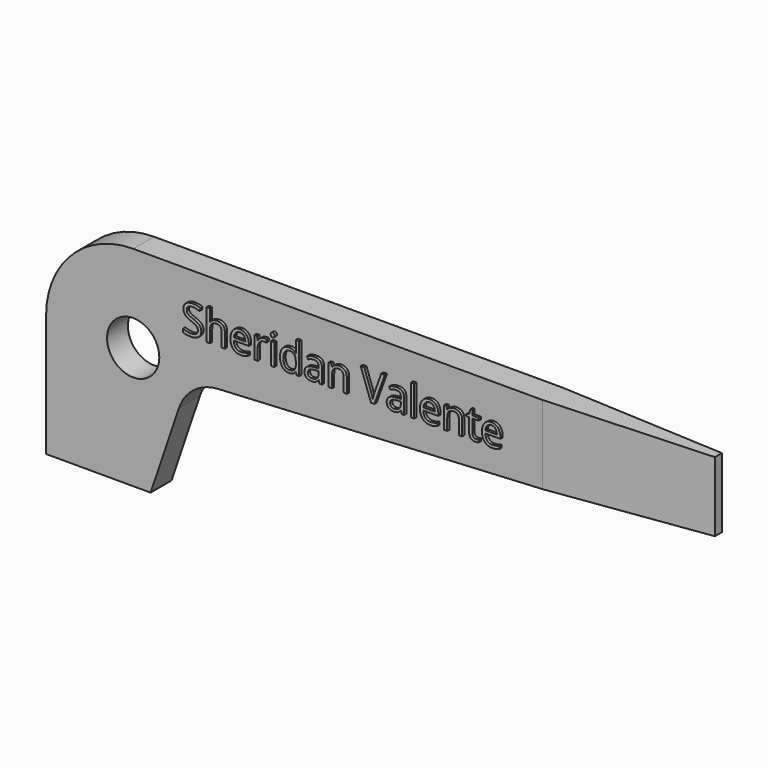
from build123d import *

# Parameters (mm, degrees)
F1_DEPTH     = 2.38125
F2_R         = 2.38125
F3_DEPTH     = 2.38225
F5_DEPTH     = 19.051
F6_TEXT_SIZE = 3.6996634056
F7_DEPTH     = 0.254


# Not quite as in the source:
# - Text() gives the source's letters only with a copy of the font that has no kerning and outlines rounded to 1/6400 em; it was checked with that copy


with BuildPart() as f1:
    # F0 (on Front) → F1 (new body)
    with BuildSketch(Plane.XZ):
        with BuildLine():
            Line((60.325, 19.05), (7.9375, 19.05))
            ThreePointArc((7.9375, 19.05), (2.3248399243, 16.7251600757), (0, 11.1125))
            Line((0, 11.1125), (0, 0))
            Line((0, 0), (9.525, 0))
            Line((9.525, 0), (12.1103451907, 7.6262422093))
            ThreePointArc((12.1103451907, 7.6262422093), (13.4737562991, 9.5178776332), (15.6634210502, 10.3194652484))
            Line((15.6634210502, 10.3194652484), (60.325, 12.7))
            Line((60.325, 12.7), (60.325, 19.05))
        make_face()
    extrude(amount=F1_DEPTH)

    # F2 (on face) → F3 (cut, through all)
    with BuildSketch(Plane.XZ.offset(2.38125)):
        with Locations((7.9375, 11.1125)):
            Circle(F2_R)
    extrude(amount=-F3_DEPTH, mode=Mode.SUBTRACT)

    # F4 (on face) → F5 (cut, through all)
    with BuildSketch(Plane.XY.offset(19.05)):
        Polygon((60.325, 0), (45.24375, 0), (60.325, -0.79375), align=None)
        Polygon((60.325, -2.38125), (60.325, -1.59385), (45.2374, -2.38125), align=None)
    extrude(amount=-F5_DEPTH, mode=Mode.SUBTRACT)

    # F6 (on face) → F7 (join)
    with BuildSketch(Plane.XZ.offset(2.38125)):
        with Locations((12.4943582341, 13.9126423746)):
            Text('Sheridan Valente', F6_TEXT_SIZE, font='Open Sans', text_align=(TextAlign.LEFT, TextAlign.BOTTOM))
    extrude(amount=F7_DEPTH)


solid = f1.part
